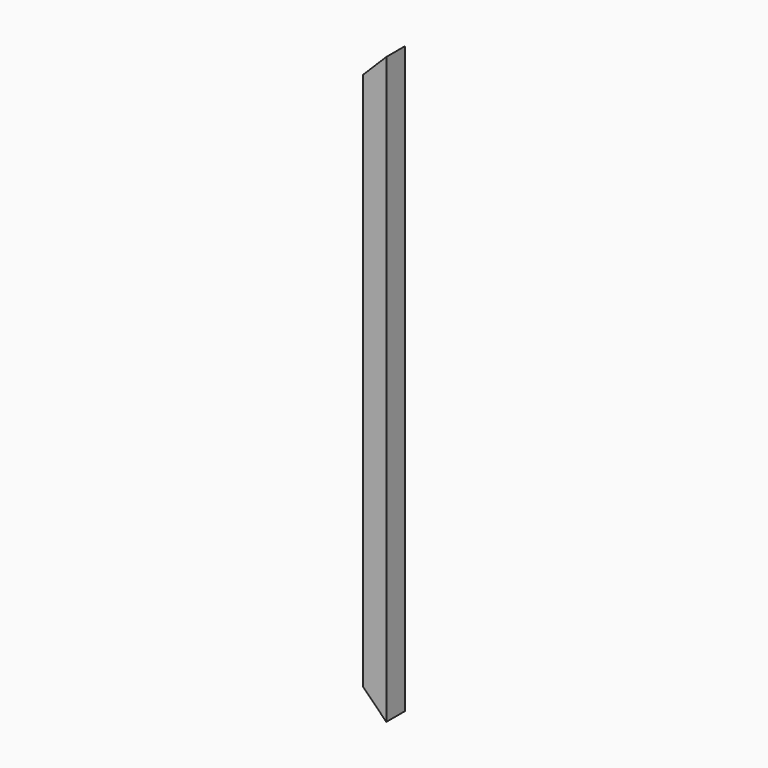
from build123d import *

# Parameters (mm, degrees)
F0_W        = 50
F0_H        = 50
F0_W_2      = 44
F0_H_2      = 44
F1_DEPTH    = 1250
F2_T1_DEPTH = 307.1682987966


# Not quite as in the source:
# - a fillet or chamfer that OpenCascade refuses, or shapes differently, is made with other operations: its cross-section is extruded or revolved along the edge and cut away or added


with BuildPart() as f1:
    # F0 (on Top) → F1 (new body)
    with BuildSketch(Plane.XY):
        with Locations((25, 25)):
            Rectangle(F0_W, F0_H)
        with Locations((25, 25)):
            Rectangle(F0_W_2, F0_H_2, mode=Mode.SUBTRACT)
    extrude(amount=F1_DEPTH)

    # F2: chamfer of 50 on 2 edges, made by hand

    # F2_s2 → F2_t1 (cut)
    with BuildSketch(Plane.XZ.offset(-178.5841493983)):
        Polygon((0, 50), (50, 0), (0, 0), align=None)
        Polygon((0, 1200), (50, 1250), (0, 1250), align=None)
    extrude(amount=F2_T1_DEPTH, mode=Mode.SUBTRACT)


solid = f1.part
